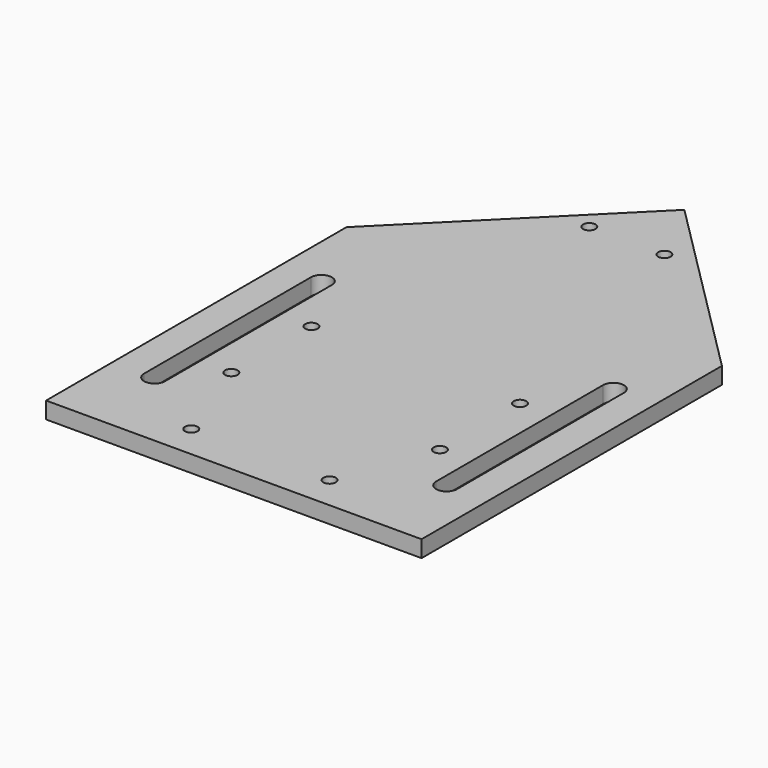
from build123d import *

# Parameters (mm, degrees)
F0_W     = 45
F0_H     = 135
F1_DEPTH = 4
F2_SIZE  = 44.99999
F5_DEPTH = 39.1207225621
F7_D     = 3
F9_D     = 3
F11_D    = 3
F14_D    = 3


# Not quite as in the source:
# - a fillet or chamfer is up to 0.001 mm smaller than in the source, because OpenCascade refuses the exact size


with BuildPart() as f1:
    # F0 (on Top) → F1 (new body)
    with BuildSketch(Plane.XY):
        with Locations((22.5, 67.5)):
            Rectangle(F0_W, F0_H)
    extrude(amount=F1_DEPTH)

    # F2 (size 45 in the source; OpenCascade refuses exactly that, so slightly less here)
    f2_edges = [f1.edges().sort_by_distance(p)[0] for p in [
        (45, 135, 2),
    ]]
    chamfer(f2_edges, length=F2_SIZE)

    # F4 (on face) → F5 (cut)
    with BuildSketch(Plane.XY.offset(4)):
        with BuildLine():
            ThreePointArc((32.5, 20), (35, 17.5), (37.5, 20))
            Line((37.5, 20), (37.5, 70))
            ThreePointArc((37.5, 70), (35, 72.5), (32.5, 70))
            Line((32.5, 70), (32.5, 20))
        make_face()
    extrude(amount=-F5_DEPTH, mode=Mode.SUBTRACT)

    # F7 (through all)
    with Locations(Plane.XY.offset(4)):
        with Locations((16.5778252002, 7.9720381196)):
            Hole(F7_D / 2)

    # F9 (through all)
    with Locations(Plane.XY.offset(4)):
        with Locations((25, 30.5)):
            Hole(F9_D / 2)

    # F11 (through all)
    with Locations(Plane.XY.offset(4)):
        with Locations((25, 54.5)):
            Hole(F11_D / 2)

    # F12: F1 across plane


with BuildPart() as f1_1:
    add(f1.part)
    add(f1.part.mirror(Plane.YZ))

    # F14 (through all)
    with Locations(Plane.XY.offset(4)):
        with Locations((-9.6168344989, 118.5341477394), (8.3831655011, 118.5341477394)):
            Hole(F14_D / 2)


solid = f1_1.part
